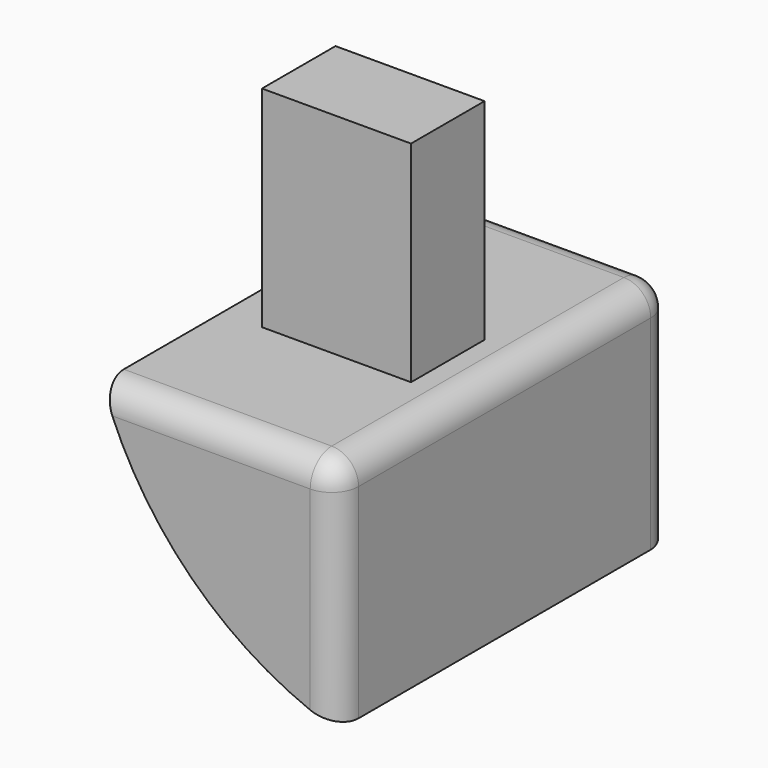
from build123d import *

# Parameters (mm, degrees)
F0_W        = 47.8054173291
F0_H        = 43.6823405325
F1_DEPTH    = 79.23727
F2_T1_DEPTH = 403.639522146
F3_R        = 5.08
F4_W        = 28.1929401681
F4_H        = 17.383787781
F5_DEPTH    = 83.42686


# Not quite as in the source:
# - a fillet or chamfer that OpenCascade refuses, or shapes differently, is made with other operations: its cross-section is extruded or revolved along the edge and cut away or added


with BuildPart() as f1:
    # F0 (on Front) → F1 (new body)
    with BuildSketch(Plane.XZ):
        with Locations((2.172973007, 21.8411702663)):
            Rectangle(F0_W, F0_H)
    extrude(amount=F1_DEPTH)

    # F2: fillet of radius 67.9298616849 on 1 edges, made by hand

    # F2_s2 → F2_t1 (cut)
    with BuildSketch(Plane.XZ.offset(-162.201126073)):
        with BuildLine():
            ThreePointArc((-21.7297356576, 64.8804504292), (-8.4877009093, 24.5851939655), (26.0756816715, 0))
            Line((26.0756816715, 0), (-21.7297356576, 0))
            Line((-21.7297356576, 0), (-21.7297356576, 64.8804504292))
        make_face()
    extrude(amount=F2_T1_DEPTH, mode=Mode.SUBTRACT)

    # F3
    f3_edges = [f1.edges().sort_by_distance(p)[0] for p in [
        (26.075682, -39.618635, 43.682341),
        (3.869087, -79.23727, 43.682341),
        (26.075682, -79.23727, 21.84117),
        (26.075682, 0, 21.84117),
        (3.869087, 0, 43.682341),
    ]]
    fillet(f3_edges, radius=F3_R)

    # F4 (on Top) → F5 (join)
    with BuildSketch(Plane.XY):
        with Locations((3.2873195596, -42.192241177)):
            Rectangle(F4_W, F4_H)
    extrude(amount=F5_DEPTH)


solid = f1.part
